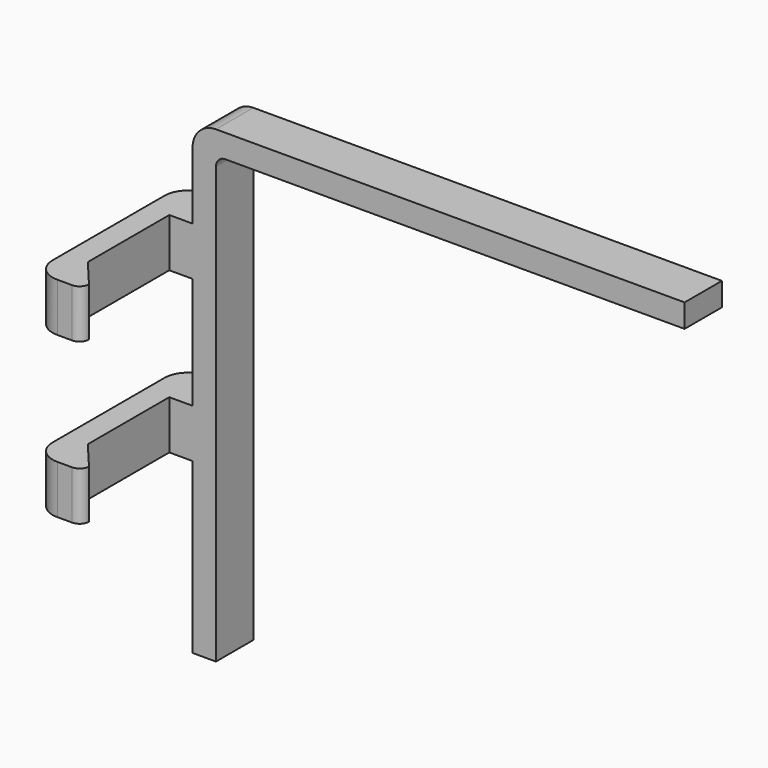
from build123d import *

# Parameters (mm, degrees)
F1_DEPTH = 10
F2_W     = 5
F2_H     = 10.4262067128
F3_DEPTH = 30
F4_R     = 4.99999
F6_DEPTH = 10.4262067128
F8_DEPTH = 10.4262067128


# Not quite as in the source:
# - a fillet or chamfer is up to 0.001 mm smaller than in the source, because OpenCascade refuses the exact size


with BuildPart() as f1:
    # F0 (on Front) → F1 (new body)
    with BuildSketch(Plane.XZ):
        with BuildLine():
            Line((-5, -51.3071772588), (0, -51.3071772588))
            Line((0, -51.3071772588), (0, 42.0990820395))
            ThreePointArc((0, 42.0990820395), (0.5857864376, 43.5132956019), (2, 44.0990820395))
            Line((2, 44.0990820395), (100.4062592983, 44.0990820395))
            Line((100.4062592983, 44.0990820395), (100.4062592983, 49.0990820395))
            Line((100.4062592983, 49.0990820395), (0, 49.0990820395))
            ThreePointArc((0, 49.0990820395), (-3.5355339059, 47.6346159455), (-5, 44.0990820395))
            Line((-5, 44.0990820395), (-5, 29.6768955886))
            Line((-5, 29.6768955886), (-15, 29.6768955886))
            Line((-15, 29.6768955886), (-15, 19.2506888759))
            Line((-15, 19.2506888759), (-5, 19.2506888759))
            Line((-5, 19.2506888759), (-5, -4.6830929693))
            Line((-5, -4.6830929693), (-15, -4.6830929693))
            Line((-15, -4.6830929693), (-15, -15.1092996821))
            Line((-15, -15.1092996821), (-5, -15.1092996821))
            Line((-5, -15.1092996821), (-5, -51.3071772588))
        make_face()
    extrude(amount=F1_DEPTH)

    # F2 (on face) → F3 (join)
    with BuildSketch(Plane.XZ.offset(10)):
        with Locations((-12.5, 24.4637922322)):
            Rectangle(F2_W, F2_H)
        with Locations((-12.5, -9.8961963257)):
            Rectangle(F2_W, F2_H)
    extrude(amount=F3_DEPTH)

    # F4 (radius 5 in the source; OpenCascade refuses exactly that, so slightly less here)
    f4_edges = [f1.edges().sort_by_distance(p)[0] for p in [
        (-15, -40, 24.463792),
        (-15, -40, -9.896196),
        (-15, 0, 24.463792),
        (-15, 0, -9.896196),
    ]]
    fillet(f4_edges, radius=F4_R)

    # F5 (on face) → F6 (join, through all)
    with BuildSketch(Plane(origin=(0, 0, -15.1092996821), x_dir=(1, 0, 0), z_dir=(0, 0, -1))):
        with BuildLine():
            Line((-6.8065949231, 40), (-10, 40))
            Line((-10, 40), (-10, 31.8107408419))
            Line((-10, 31.8107408419), (-4.8065949231, 38))
            ThreePointArc((-4.8065949231, 38), (-5.3923813608, 39.4142135624), (-6.8065949231, 40))
        make_face()
    extrude(amount=-F6_DEPTH)

    # F7 (on face) → F8 (join, through all)
    with BuildSketch(Plane(origin=(0, 0, 19.2506888759), x_dir=(1, 0, 0), z_dir=(0, 0, -1))):
        with BuildLine():
            Line((-6.8065949231, 40), (-10, 40))
            Line((-10, 40), (-10, 31.8107408419))
            Line((-10, 31.8107408419), (-4.8065949231, 38))
            ThreePointArc((-4.8065949231, 38), (-5.3923813608, 39.4142135624), (-6.8065949231, 40))
        make_face()
    extrude(amount=-F8_DEPTH)


solid = f1.part
